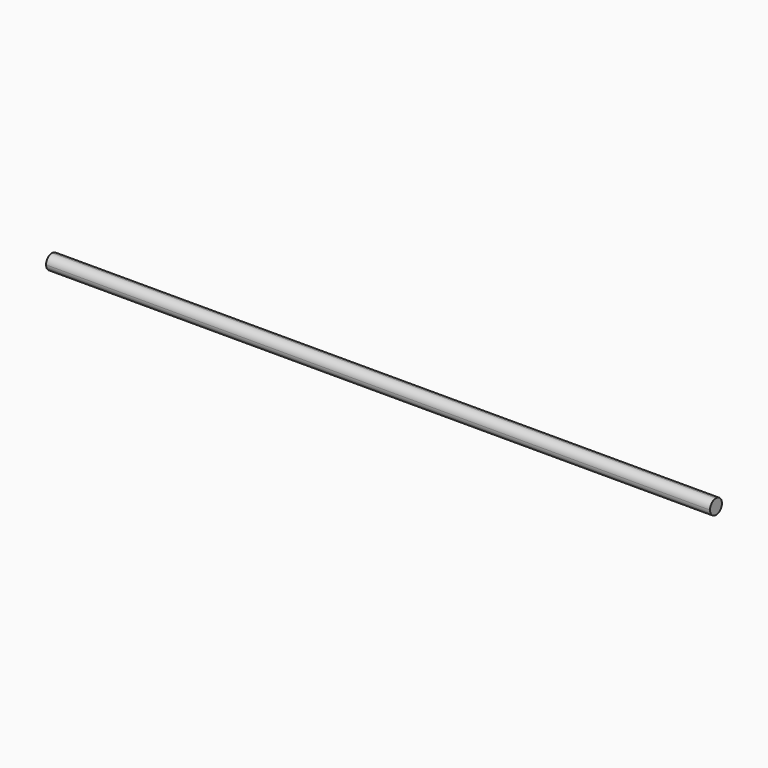
from build123d import *

# Parameters (mm, degrees)
F0_W     = 670
F0_H     = 15
F1_DEPTH = 7.5
F2_R     = 7.49999


# Not quite as in the source:
# - a fillet or chamfer is up to 0.001 mm smaller than in the source, because OpenCascade refuses the exact size


with BuildPart() as f1:
    # F0 (on Front) → F1 (new body, symmetric)
    with BuildSketch(Plane.XZ):
        Rectangle(F0_W, F0_H)
    extrude(amount=F1_DEPTH, both=True)

    # F2 (radius 7.5 in the source; OpenCascade refuses exactly that, so slightly less here)
    f2_edges = [f1.edges().sort_by_distance(p)[0] for p in [
        (0, 7.5, -7.5),
        (0, -7.5, -7.5),
        (0, -7.5, 7.5),
        (0, 7.5, 7.5),
    ]]
    fillet(f2_edges, radius=F2_R)


solid = f1.part
